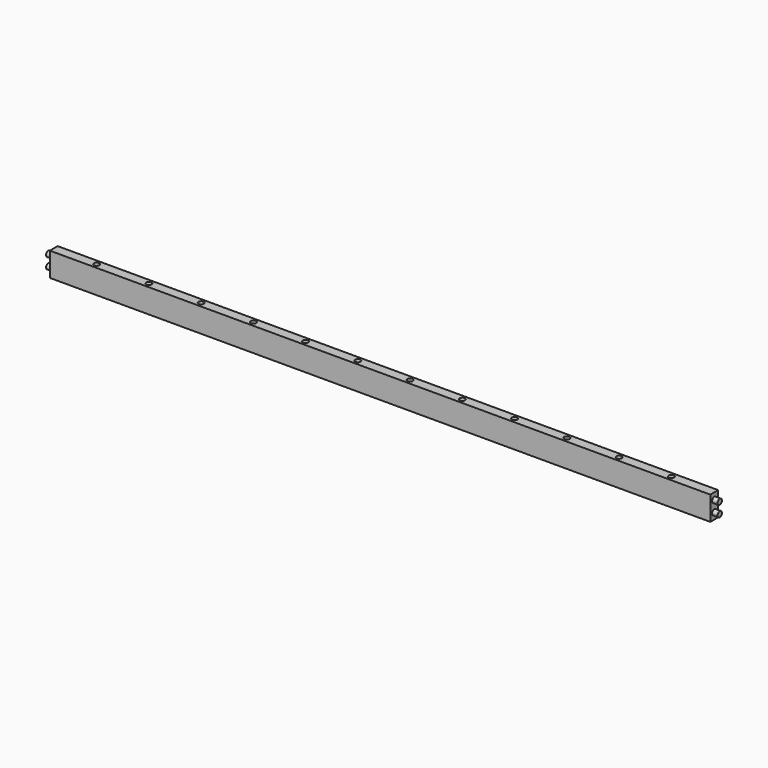
from build123d import *

# Parameters (mm, degrees)
F0_W          = 1210
F0_H          = 18
F1_DEPTH      = 44
F2_R          = 5
F3_DEPTH      = 10
F3_DEPTH_BACK = 1220
F4_R          = 5
F5_DEPTH      = 10


# Not quite as in the source:
# - a feature names something its author has since deleted; it is built from what else it names


with BuildPart() as f1:
    # F0 (on Top) → F1 (new body)
    with BuildSketch(Plane.XY):
        with Locations((605, 9)):
            Rectangle(F0_W, F0_H)
    extrude(amount=F1_DEPTH)

    # F2 (on face) → F3 (join, two sides)
    with BuildSketch(Plane(origin=(0, 0, 0), x_dir=(0, -1, 0), z_dir=(-1, 0, 0))) as f3_sk:
        with Locations((-9, 32)):
            Circle(F2_R)
        with Locations((-9, 12)):
            Circle(F2_R)
    extrude(amount=F3_DEPTH)
    extrude(f3_sk.sketch, amount=-F3_DEPTH_BACK)

    # F4 (on face) → F5 (cut)
    with BuildSketch(Plane.XY.offset(44)):
        with Locations((78.65, 9)):
            Circle(F4_R)
        with Locations((174.35, 9)):
            Circle(F4_R)
        with Locations((270.05, 9)):
            Circle(F4_R)
        with Locations((365.75, 9)):
            Circle(F4_R)
        with Locations((461.45, 9)):
            Circle(F4_R)
        with Locations((557.15, 9)):
            Circle(F4_R)
        with Locations((652.85, 9)):
            Circle(F4_R)
        with Locations((748.55, 9)):
            Circle(F4_R)
        with Locations((844.25, 9)):
            Circle(F4_R)
        with Locations((939.95, 9)):
            Circle(F4_R)
        with Locations((1035.65, 9)):
            Circle(F4_R)
        with Locations((1131.35, 9)):
            Circle(F4_R)
    extrude(amount=-F5_DEPTH, mode=Mode.SUBTRACT)


solid = f1.part
